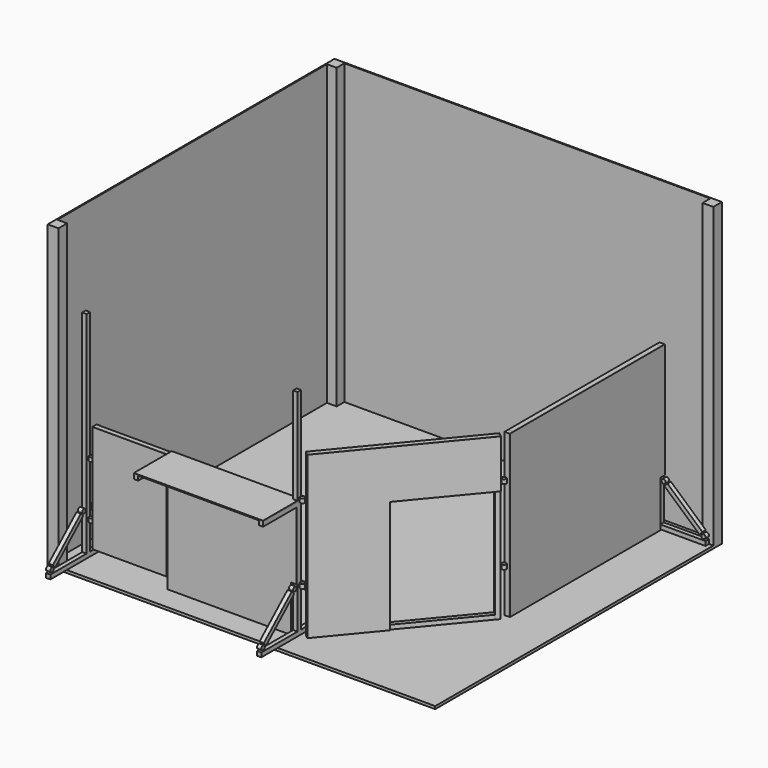
from build123d import *

# Parameters (mm, degrees)
F0_W           = 3600
F0_H           = 3330
F1_DEPTH       = 25
F2_W           = 10
F2_H           = 3130
F2_W_2         = 3400
F2_H_2         = 10
F3_DEPTH       = 2770
F4_W           = 40
F4_H           = 40
F5_DEPTH       = 1500
F6_DEPTH       = 2000
F7_W           = 40
F7_H           = 40
F8_DEPTH       = 1720
F10_DEPTH      = 40
F9_R           = 20
F9_W           = 420
F9_H           = 40
F12_DEPTH      = 40
F11_R          = 20
F11_W          = 420
F11_H          = 40
F13_R          = 20
F14_DEPTH      = 40
F13_W          = 420
F13_H          = 40
F16_W          = 40
F16_H          = 40
F17_DEPTH      = 400
F19_R          = 20
F20_DEPTH      = 40
F22_R          = 20
F23_DEPTH      = 40
F26_DEPTH      = 1500
F27_W          = 40
F27_H          = 40
F28_DEPTH      = 1354
F29_W          = 40
F29_H          = 40
F30_DEPTH      = 1120
F31_W          = 40
F31_H          = 40
F32_DEPTH      = 1060
F32_DEPTH_BACK = 40
F33_W          = 40
F33_H          = 40
F34_DEPTH      = 400
F36_R          = 20
F37_DEPTH      = 40
F39_R          = 20
F40_DEPTH      = 40
F42_W          = 40
F42_H          = 40
F43_DEPTH      = 1000
F44_W          = 40
F44_H          = 40
F45_DEPTH      = 610
F47_DEPTH      = 10
F49_DEPTH      = 10
F51_DEPTH      = 10
F52_W          = 690
F52_H          = 1000
F53_DEPTH      = 10
F55_DEPTH      = 10


# Not quite as in the source:
# - a feature names something its author has since deleted; it is built from what else it names


with BuildPart() as f1:
    # F0 (on Top) → F1 (new body)
    with BuildSketch(Plane.XY):
        with Locations((2.8558038175, -13.8908525274)):
            Rectangle(F0_W, F0_H)
    extrude(amount=F1_DEPTH)

    # F2 (on face) → F3 (join)
    with BuildSketch(Plane.XY.offset(25)):
        Polygon((-1697.1441961825, 1651.1091474726), (-1797.1441961825, 1651.1091474726), (-1797.1441961825, 1551.1091474726), (-1787.1441961825, 1551.1091474726), (-1697.1441961825, 1551.1091474726), (-1697.1441961825, 1641.1091474726), align=None)
        Polygon((-1787.1441961825, -1578.8908525274), (-1797.1441961825, -1578.8908525274), (-1797.1441961825, -1678.8908525274), (-1697.1441961825, -1678.8908525274), (-1697.1441961825, -1578.8908525274), align=None)
        Polygon((1802.8558038175, 1651.1091474726), (1702.8558038175, 1651.1091474726), (1702.8558038175, 1641.1091474726), (1702.8558038175, 1551.1091474726), (1802.8558038175, 1551.1091474726), align=None)
        with Locations((-1792.1441961825, -13.8908525274)):
            Rectangle(F2_W, F2_H)
        with Locations((2.8558038175, 1646.1091474726)):
            Rectangle(F2_W_2, F2_H_2)
    extrude(amount=F3_DEPTH)

    # F4 (on face) → F5 (join)
    with BuildSketch(Plane.XY.offset(25)):
        with Locations((1322.8558038175, 1531.1091474726)):
            Rectangle(F4_W, F4_H)
        with Locations((1322.8558038175, -228.8908525274)):
            Rectangle(F4_W, F4_H)
    extrude(amount=F5_DEPTH)

    # F4 (on face) → F6 (join)
    with BuildSketch(Plane.XY.offset(25)):
        with Locations((-1640.5064868927, -1428.8908525274)):
            Rectangle(F4_W, F4_H)
        with Locations((319.4935131073, -1428.8908525274)):
            Rectangle(F4_W, F4_H)
    extrude(amount=F6_DEPTH)

    # F11 (on face) → F12, piece 4 (join)
    with BuildSketch(Plane.YZ.offset(-1620.5064868927)):
        with Locations((-1658.8908525274, 45)):
            Rectangle(F11_W, F11_H)
        with Locations((-1198.8908525274, 45)):
            Rectangle(F11_W, F11_H)
    extrude(amount=-F12_DEPTH)

    # F13 (on face) → F14, piece 7 (join)
    with BuildSketch(Plane.YZ.offset(339.4935131073)):
        with Locations((-1658.8908525274, 45)):
            Rectangle(F13_W, F13_H)
        with Locations((-1198.8908525274, 45)):
            Rectangle(F13_W, F13_H)
    extrude(amount=-F14_DEPTH)

    # F16 (on face) → F17 (join)
    with BuildSketch(Plane.XZ.offset(1448.8908525274)):
        with Locations((319.4935131073, 1105)):
            Rectangle(F16_W, F16_H)
    extrude(amount=F17_DEPTH)

    # F29 (on face) → F30 (join)
    with BuildSketch(Plane(origin=(299.4935131073, 0, 0), x_dir=(0, -1, 0), z_dir=(-1, 0, 0))):
        with Locations((1428.8908525274, 1105)):
            Rectangle(F29_W, F29_H)
        with Locations((1428.8908525274, 45)):
            Rectangle(F29_W, F29_H)
    extrude(amount=F30_DEPTH)

    # F31 (on face) → F32 (join, two sides)
    with BuildSketch(Plane.XY.offset(65)) as f32_sk:
        with Locations((-840.5064868927, -1428.8908525274)):
            Rectangle(F31_W, F31_H)
    extrude(amount=F32_DEPTH)
    extrude(f32_sk.sketch, amount=-F32_DEPTH_BACK)

    # F33 (on face) → F34 (join)
    with BuildSketch(Plane.XZ.offset(1448.8908525274)):
        with Locations((-840.5064868927, 1105)):
            Rectangle(F33_W, F33_H)
    extrude(amount=F34_DEPTH)


with BuildPart() as f8:
    # F7 (on face) → F8 (new body)
    with BuildSketch(Plane.XZ.offset(-1511.1091474726)):
        with Locations((1322.8558038175, 1505)):
            Rectangle(F7_W, F7_H)
    extrude(amount=F8_DEPTH)


with BuildPart() as f8b:
    # F7 (on face) → F8, piece 2 (new body)
    with BuildSketch(Plane.XZ.offset(-1511.1091474726)):
        with Locations((1322.8558038175, 45)):
            Rectangle(F7_W, F7_H)
    extrude(amount=F8_DEPTH)


with BuildPart() as f10:
    # F9 (on face) → F10 (new body)
    with BuildSketch(Plane.XZ.offset(-1511.1091474726)):
        Polygon((911.9323699124, 129.8943540981), (938.5569637907, 100.0425367194), (1263.7792377226, 390.1056459019), (1237.1546438443, 419.9574632806), align=None)
    extrude(amount=-F10_DEPTH)


with BuildPart() as f10b:
    # F9 (on face) → F10, piece 2 (new body)
    with BuildSketch(Plane.XZ.offset(-1511.1091474726)):
        with Locations((1272.8558038175, 425)):
            Circle(F9_R)
    extrude(amount=-F10_DEPTH)


with BuildPart() as f10c:
    # F9 (on face) → F10, piece 3 (new body)
    with BuildSketch(Plane.XZ.offset(-1511.1091474726)):
        with Locations((902.8558038175, 95)):
            Circle(F9_R)
    extrude(amount=-F10_DEPTH)


with BuildPart() as f10d:
    # F9 (on face) → F10, piece 4 (new body)
    with BuildSketch(Plane.XZ.offset(-1511.1091474726)):
        with Locations((1092.8558038175, 45)):
            Rectangle(F9_W, F9_H)
    extrude(amount=-F10_DEPTH)


with BuildPart() as f10e:
    # F9 (on face) → F10, piece 5 (new body)
    with BuildSketch(Plane.XZ.offset(-1511.1091474726)):
        with Locations((1372.8558038175, 425)):
            Circle(F9_R)
    extrude(amount=-F10_DEPTH)


with BuildPart() as f10f:
    # F9 (on face) → F10, piece 6 (new body)
    with BuildSketch(Plane.XZ.offset(-1511.1091474726)):
        Polygon((1733.7792377226, 129.8943540981), (1408.5569637907, 419.9574632806), (1381.9323699124, 390.1056459019), (1707.1546438443, 100.0425367194), align=None)
    extrude(amount=-F10_DEPTH)


with BuildPart() as f10g:
    # F9 (on face) → F10, piece 7 (new body)
    with BuildSketch(Plane.XZ.offset(-1511.1091474726)):
        with Locations((1742.8558038175, 95)):
            Circle(F9_R)
    extrude(amount=-F10_DEPTH)


with BuildPart() as f10h:
    # F9 (on face) → F10, piece 8 (new body)
    with BuildSketch(Plane.XZ.offset(-1511.1091474726)):
        with Locations((1552.8558038175, 45)):
            Rectangle(F9_W, F9_H)
    extrude(amount=-F10_DEPTH)


with BuildPart() as f12:
    # F11 (on face) → F12 (new body)
    with BuildSketch(Plane.YZ.offset(-1620.5064868927)):
        Polygon((-1839.8142864325, 129.8943540981), (-1813.1896925542, 100.0425367194), (-1487.9674186223, 390.1056459019), (-1514.5920125006, 419.9574632806), align=None)
    extrude(amount=-F12_DEPTH)


with BuildPart() as f12b:
    # F11 (on face) → F12, piece 2 (new body)
    with BuildSketch(Plane.YZ.offset(-1620.5064868927)):
        with Locations((-1478.8908525274, 425)):
            Circle(F11_R)
    extrude(amount=-F12_DEPTH)


with BuildPart() as f12c:
    # F11 (on face) → F12, piece 3 (new body)
    with BuildSketch(Plane.YZ.offset(-1620.5064868927)):
        with Locations((-1848.8908525274, 95)):
            Circle(F11_R)
    extrude(amount=-F12_DEPTH)


with BuildPart() as f12d:
    # F11 (on face) → F12, piece 5 (new body)
    with BuildSketch(Plane.YZ.offset(-1620.5064868927)):
        with Locations((-1008.8908525274, 95)):
            Circle(F11_R)
    extrude(amount=-F12_DEPTH)


with BuildPart() as f12e:
    # F11 (on face) → F12, piece 6 (new body)
    with BuildSketch(Plane.YZ.offset(-1620.5064868927)):
        Polygon((-1017.9674186223, 129.8943540981), (-1343.1896925542, 419.9574632806), (-1369.8142864325, 390.1056459019), (-1044.5920125006, 100.0425367194), align=None)
    extrude(amount=-F12_DEPTH)


with BuildPart() as f12f:
    # F11 (on face) → F12, piece 7 (new body)
    with BuildSketch(Plane.YZ.offset(-1620.5064868927)):
        with Locations((-1378.8908525274, 425)):
            Circle(F11_R)
    extrude(amount=-F12_DEPTH)


with BuildPart() as f14:
    # F13 (on face) → F14 (new body)
    with BuildSketch(Plane.YZ.offset(339.4935131073)):
        with Locations((-1848.8908525274, 95)):
            Circle(F13_R)
    extrude(amount=-F14_DEPTH)


with BuildPart() as f14b:
    # F13 (on face) → F14, piece 2 (new body)
    with BuildSketch(Plane.YZ.offset(339.4935131073)):
        Polygon((-1839.8142864325, 129.8943540981), (-1813.1896925542, 100.0425367194), (-1487.9674186223, 390.1056459019), (-1514.5920125006, 419.9574632806), align=None)
    extrude(amount=-F14_DEPTH)


with BuildPart() as f14c:
    # F13 (on face) → F14, piece 3 (new body)
    with BuildSketch(Plane.YZ.offset(339.4935131073)):
        with Locations((-1478.8908525274, 425)):
            Circle(F13_R)
    extrude(amount=-F14_DEPTH)


with BuildPart() as f14d:
    # F13 (on face) → F14, piece 4 (new body)
    with BuildSketch(Plane.YZ.offset(339.4935131073)):
        with Locations((-1378.8908525274, 425)):
            Circle(F13_R)
    extrude(amount=-F14_DEPTH)


with BuildPart() as f14e:
    # F13 (on face) → F14, piece 5 (new body)
    with BuildSketch(Plane.YZ.offset(339.4935131073)):
        Polygon((-1017.9674186223, 129.8943540981), (-1343.1896925542, 419.9574632806), (-1369.8142864325, 390.1056459019), (-1044.5920125006, 100.0425367194), align=None)
    extrude(amount=-F14_DEPTH)


with BuildPart() as f14f:
    # F13 (on face) → F14, piece 6 (new body)
    with BuildSketch(Plane.YZ.offset(339.4935131073)):
        with Locations((-1008.8908525274, 95)):
            Circle(F13_R)
    extrude(amount=-F14_DEPTH)


with BuildPart() as f20:
    # F19 (on offset) → F20 (new body)
    with BuildSketch(Plane.XY.offset(425)):
        with Locations((1322.8558038175, -278.8908525274)):
            Circle(F19_R)
    extrude(amount=F20_DEPTH)


with BuildPart() as f20b:
    # F19 (on offset) → F20, piece 2 (new body)
    with BuildSketch(Plane.XY.offset(425)):
        with Locations((369.4935131073, -1428.8908525274)):
            Circle(F19_R)
    extrude(amount=F20_DEPTH)


with BuildPart() as f23:
    # F22 (on offset) → F23 (new body)
    with BuildSketch(Plane.XY.offset(1125)):
        with Locations((1322.8558038175, -278.8908525274)):
            Circle(F22_R)
    extrude(amount=F23_DEPTH)


with BuildPart() as f23b:
    # F22 (on offset) → F23, piece 2 (new body)
    with BuildSketch(Plane.XY.offset(1125)):
        with Locations((369.4935131073, -1428.8908525274)):
            Circle(F22_R)
    extrude(amount=F23_DEPTH)


with BuildPart() as f26:
    # F25 (on offset) → F26 (new body)
    with BuildSketch(Plane.XY.offset(25)):
        Polygon((1288.3121452678, -289.2221474123), (1262.783411151, -320.0163633367), (1293.5776270754, -345.5450974534), (1319.1063611921, -314.7508815291), align=None)
    extrude(amount=F26_DEPTH)


with BuildPart() as f26b:
    # F25 (on offset) → F26, piece 2 (new body)
    with BuildSketch(Plane.XY.offset(25)):
        Polygon((373.2429557327, -1393.0308235258), (404.037171657, -1418.5595576425), (429.5659057738, -1387.7653417182), (398.7716898494, -1362.2366076014), align=None)
    extrude(amount=F26_DEPTH)


with BuildPart() as f28:
    # F27 (on face) → F28 (new body)
    with BuildSketch(Plane(origin=(357.1247955866, 430.7843082598, 0), x_dir=(0.7698553981, -0.6382183529, 0), z_dir=(-0.6382183529, -0.7698553981, 0))):
        with Locations((1196.4009420328, 1505)):
            Rectangle(F27_W, F27_H)
    extrude(amount=F28_DEPTH)


with BuildPart() as f28b:
    # F27 (on face) → F28, piece 2 (new body)
    with BuildSketch(Plane(origin=(357.1247955866, 430.7843082598, 0), x_dir=(0.7698553981, -0.6382183529, 0), z_dir=(-0.6382183529, -0.7698553981, 0))):
        with Locations((1196.4009420328, 45)):
            Rectangle(F27_W, F27_H)
    extrude(amount=F28_DEPTH)


with BuildPart() as f37:
    # F36 (on offset) → F37 (new body)
    with BuildSketch(Plane.XY.offset(325)):
        with Locations((-1590.5064868927, -1428.8908525274)):
            Circle(F36_R)
    extrude(amount=F37_DEPTH)


with BuildPart() as f40:
    # F39 (on offset) → F40 (new body)
    with BuildSketch(Plane.XY.offset(825)):
        with Locations((-1590.5064868927, -1428.8908525274)):
            Circle(F39_R)
    extrude(amount=F40_DEPTH)


with BuildPart() as f43:
    # F42 (on offset) → F43 (new body)
    with BuildSketch(Plane.XY.offset(125)):
        with Locations((-1540.5064868927, -1427.1560311317)):
            Rectangle(F42_W, F42_H)
    extrude(amount=F43_DEPTH)


with BuildPart() as f43b:
    # F42 (on offset) → F43, piece 2 (new body)
    with BuildSketch(Plane.XY.offset(125)):
        with Locations((-890.5064868927, -1428.8908525274)):
            Rectangle(F42_W, F42_H)
    extrude(amount=F43_DEPTH)


with BuildPart() as f45:
    # F44 (on face) → F45 (new body)
    with BuildSketch(Plane(origin=(-910.5064868927, 0, 0), x_dir=(0, -1, 0), z_dir=(-1, 0, 0))):
        with Locations((1428.8908525274, 1105)):
            Rectangle(F44_W, F44_H)
    extrude(amount=F45_DEPTH)


with BuildPart() as f45b:
    # F44 (on face) → F45, piece 2 (new body)
    with BuildSketch(Plane(origin=(-910.5064868927, 0, 0), x_dir=(0, -1, 0), z_dir=(-1, 0, 0))):
        with Locations((1428.8908525274, 145)):
            Rectangle(F44_W, F44_H)
    extrude(amount=F45_DEPTH)


with BuildPart() as f47:
    # F46 (on face) → F47 (new body)
    with BuildSketch(Plane.YZ.offset(1342.8558038175)):
        Polygon((1550.4523486232, 1525), (-249.5476513768, 1525), (-249.5476513768, 25), (1500.4523486232, 25), (1500.4523486232, 455), (1550.4523486232, 455), align=None)
    extrude(amount=F47_DEPTH)


with BuildPart() as f49:
    # F48 (on face) → F49 (new body)
    with BuildSketch(Plane(origin=(936.4528314888, -776.3294057132, 0), x_dir=(0.6382183529, 0.7698553981, 0), z_dir=(0.7698553981, -0.6382183529, 0))):
        Polygon((599.8120307922, 1525), (-834.2217947771, 1525), (-834.2217947771, 25), (-220.1879692078, 25), (-220.1879692078, 1075), (599.8120307922, 1075), align=None)
    extrude(amount=F49_DEPTH)


with BuildPart() as f51:
    # F50 (on face) → F51 (new body)
    with BuildSketch(Plane.XZ.offset(1448.8908525274)):
        Polygon((299.8368442059, 1125), (-820.5064868927, 1125), (-820.5064868927, 1085), (-860.0699305534, 1085), (-860.0699305534, 65.1121363044), (-860.0699305534, 24.4796648622), (-820.5064868927, 24.4796648622), (287.693721056, 24.4796648622), (287.693721056, 454.4796648622), (337.693721056, 454.4796648622), (337.693721056, 1085), (299.8368442059, 1085), align=None)
    extrude(amount=F51_DEPTH)


with BuildPart() as f53:
    # F52 (on face) → F53 (new body)
    with BuildSketch(Plane.XZ.offset(1447.1560311317)):
        with Locations((-1215.5064868927, 625)):
            Rectangle(F52_W, F52_H)
    extrude(amount=F53_DEPTH)


with BuildPart() as f55:
    # F54 (on face) → F55 (new body)
    with BuildSketch(Plane.XY.offset(1125)):
        Polygon((299.4935131073, -1408.8908525274), (-860.5064868927, -1408.8908525274), (-860.5064868927, -1848.8991260529), (339.4720256329, -1848.8991260529), (339.4720256329, -1448.8908525274), (299.4935131073, -1448.8908525274), align=None)
    extrude(amount=F55_DEPTH)


solid = Compound([f1.part, f8.part, f8b.part, f10.part, f10b.part, f10c.part, f10d.part, f10e.part, f10f.part, f10g.part, f10h.part, f12.part, f12b.part, f12c.part, f12d.part, f12e.part, f12f.part, f14.part, f14b.part, f14c.part, f14d.part, f14e.part, f14f.part, f20.part, f20b.part, f23.part, f23b.part, f26.part, f26b.part, f28.part, f28b.part, f37.part, f40.part, f43.part, f43b.part, f45.part, f45b.part, f47.part, f49.part, f51.part, f53.part, f55.part])
